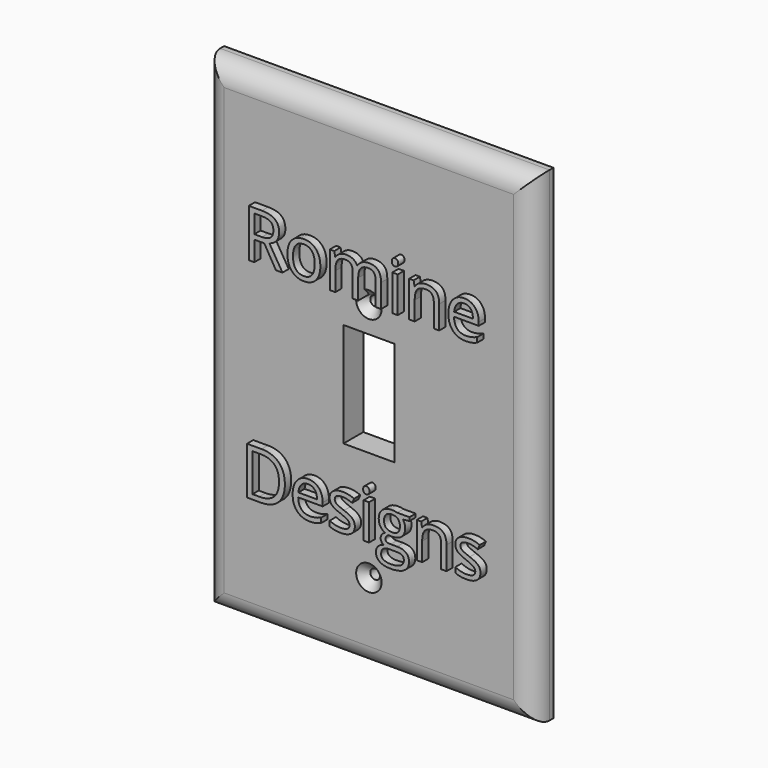
from build123d import *

# Parameters (mm, degrees)
F0_W           = 84.1375
F0_H           = 123.825
F1_DEPTH       = 6.35
F2_R           = 5.08
F3_TEXT_SIZE   = 17.1321392473
F3_TEXT_SIZE_2 = 16.9700477272
F4_DEPTH       = 2


# Not quite as in the source:
# - a fillet or chamfer that OpenCascade refuses, or shapes differently, is made with other operations: its cross-section is extruded or revolved along the edge and cut away or added
# - a feature names something its author has since deleted; it is built from what else it names
# - Text() gives the source's letters only with a copy of the font that has no kerning and outlines rounded to 1/6400 em; it was checked with that copy


with BuildPart() as f1:
    # F0 (on Front) → F1 (new body)
    with BuildSketch(Plane.XZ):
        Rectangle(F0_W, F0_H)
        with BuildLine():
            ThreePointArc((1.25, -41.4125), (-0.8838834765, -42.2963834765), (0, -40.1625))
            ThreePointArc((0, -40.1625), (0.8838834765, -40.5286165235), (1.25, -41.4125))
        make_face(mode=Mode.SUBTRACT)
        Polygon((-6.4975055866, -13.3328922093), (-6.4975055866, 13.3328922093), (0, 13.3328922093), (6.4975055866, 13.3328922093), (6.4975055866, -13.3328922093), (0, -13.3328922093), align=None, mode=Mode.SUBTRACT)
        with BuildLine():
            ThreePointArc((1.25, 20.0275), (0.8838834765, 19.1436165235), (0, 18.7775))
            ThreePointArc((0, 18.7775), (-0.8838834765, 20.9113834765), (1.25, 20.0275))
        make_face(mode=Mode.SUBTRACT)
    extrude(amount=F1_DEPTH)

    # F2
    f2_edges = [f1.edges().sort_by_distance(p)[0] for p in [
        (-42.06875, -6.35, 0),
        (42.06875, -6.35, 0),
        (0, -6.35, -61.9125),
        (0, -6.35, 61.9125),
    ]]
    fillet(f2_edges, radius=F2_R)

    # F3 (on face) → F4 (join)
    with BuildSketch(Plane.XZ.offset(6.35)):
        with Locations((-30.7749435714, 21.3723704219)):
            Text('Romine', F3_TEXT_SIZE, font='Open Sans', text_align=(TextAlign.LEFT, TextAlign.BOTTOM))
        with Locations((-31.2050010434, -32.1627836674)):
            Text('Designs', F3_TEXT_SIZE_2, font='Open Sans', text_align=(TextAlign.LEFT, TextAlign.BOTTOM))
    extrude(amount=F4_DEPTH)

    # F5: chamfer of 2 on 2 edges, made by hand


with BuildPart() as f5_tool1:
    # F5_s2 → F5_t3 (revolve)
    with BuildSketch(Plane.XY.offset(20.0275)):
        Polygon((3.25, -6.35), (1.25, -4.35), (1.25, -6.35), align=None)
    revolve(axis=Axis((0, -6.35, 20.0275), (0, -1, 0)))

    split(bisect_by=Plane.XY.offset(21.3723704219), keep=Keep.BOTTOM)

    split(bisect_by=Plane.YZ.offset(-1.1363426735), keep=Keep.TOP)


with BuildPart() as f5_tool6:
    # F5_s7 → F5_t8 (revolve)
    with BuildSketch(Plane.XY.offset(20.0275)):
        Polygon((3.25, -6.35), (1.25, -4.35), (1.25, -6.35), align=None)
    revolve(axis=Axis((0, -6.35, 20.0275), (0, -1, 0)))

    split(bisect_by=Plane.YZ.offset(-2.5256520906), keep=Keep.TOP)

    split(bisect_by=Plane.XY.offset(21.3723704219), keep=Keep.BOTTOM)

    split(bisect_by=Plane.YZ.offset(-1.1363426735), keep=Keep.BOTTOM)


with BuildPart() as f5_tool12:
    # F5_s13 → F5_t14 (revolve)
    with BuildSketch(Plane.XY.offset(20.0275)):
        Polygon((3.25, -6.35), (1.25, -4.35), (1.25, -6.35), align=None)
    revolve(axis=Axis((0, -6.35, 20.0275), (0, -1, 0)))

    split(bisect_by=Plane.XY.offset(21.3723704219), keep=Keep.TOP)

    split(bisect_by=Plane.YZ.offset(-1.1363426735), keep=Keep.TOP)


with BuildPart() as f5_tool17:
    # F5_s18 → F5_t19 (revolve)
    with BuildSketch(Plane.XY.offset(20.0275)):
        Polygon((3.25, -6.35), (1.25, -4.35), (1.25, -6.35), align=None)
    revolve(axis=Axis((0, -6.35, 20.0275), (0, -1, 0)))

    split(bisect_by=Plane.YZ.offset(-2.5256520906), keep=Keep.BOTTOM)

    split(bisect_by=Plane.XY.offset(21.3723704219), keep=Keep.BOTTOM)


with BuildPart() as f5_tool22:
    # F5_s23 → F5_t24 (revolve)
    with BuildSketch(Plane.XY.offset(20.0275)):
        Polygon((3.25, -6.35), (1.25, -4.35), (1.25, -6.35), align=None)
    revolve(axis=Axis((0, -6.35, 20.0275), (0, -1, 0)))

    split(bisect_by=Plane.YZ.offset(-2.5256520906), keep=Keep.BOTTOM)

    split(bisect_by=Plane.XY.offset(21.3723704219), keep=Keep.TOP)


with BuildPart() as f5_tool27:
    # F5_s28 → F5_t29 (revolve)
    with BuildSketch(Plane.YZ):
        Polygon((-6.35, -38.1625), (-4.35, -40.1625), (-6.35, -40.1625), align=None)
    revolve(axis=Axis((0, -6.35, -41.4125), (0, -1, 0)))


with BuildPart() as f1_1:
    add(f1.part)

    # F5_t30: cut F5_tool1, F5_tool6, F5_tool12, F5_tool17, F5_tool22, F5_tool27
    add([f5_tool1.part, f5_tool6.part, f5_tool12.part, f5_tool17.part, f5_tool22.part, f5_tool27.part], mode=Mode.SUBTRACT)


solid = f1_1.part
